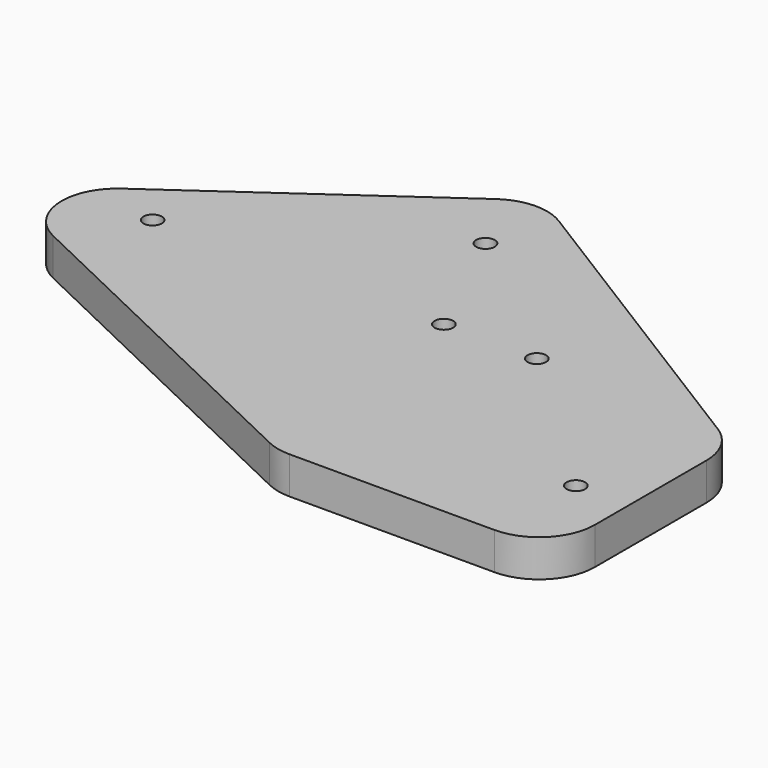
from build123d import *

# Parameters (mm, degrees)
F0_R     = 0.5
F1_DEPTH = 2
F2_R     = 3


with BuildPart() as f1:
    # F0 (on Top) → F1 (new body)
    with BuildSketch(Plane.XY):
        Polygon((-11.8603997611, -5.284095183), (2.8522056527, -5.284095183), (2.8522056527, 6.8704825826), (-17.2913148999, 19.4052960724), (-35.9591057258, 6.2361949424), align=None)
        Circle(F0_R, mode=Mode.SUBTRACT)
        with Locations((-28.9777747887, 7.7645713531)):
            Circle(F0_R, mode=Mode.SUBTRACT)
        with Locations((-16.7303260748, 14.8356391649)):
            Circle(F0_R, mode=Mode.SUBTRACT)
        with Locations((-13.5, 8)):
            Circle(F0_R, mode=Mode.SUBTRACT)
        with Locations((-8.5, 8)):
            Circle(F0_R, mode=Mode.SUBTRACT)
    extrude(amount=F1_DEPTH)

    # F2
    f2_edges = [f1.edges().sort_by_distance(p)[0] for p in [
        (-17.291315, 19.405296, 1),
        (2.852206, -5.284095, 1),
        (2.852206, 6.870483, 1),
        (-35.959106, 6.236195, 1),
        (-11.8604, -5.284095, 1),
    ]]
    fillet(f2_edges, radius=F2_R)


solid = f1.part
